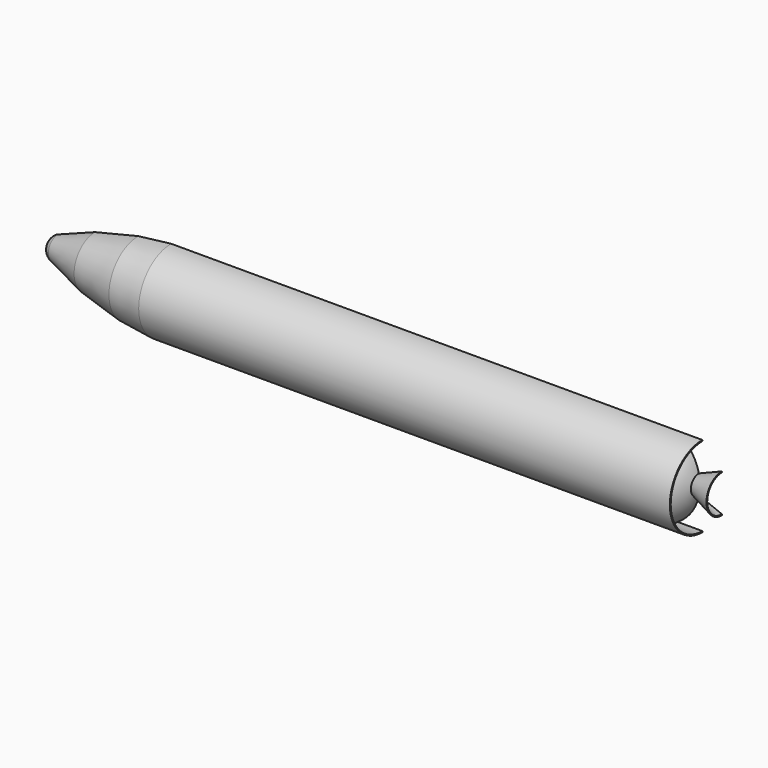
from build123d import *

# Parameters (mm, degrees)
F1_ANGLE = 180


with BuildPart() as f1:
    # F0 (on Front) → F1 (revolve)
    with BuildSketch(Plane.XZ):
        with BuildLine():
            Line((13952.3196879505, 1066.8), (0, 1066.8))
            Line((0, 1066.8), (-864.9686047513, 961.8114734625))
            Line((-864.9686047513, 961.8114734625), (-2002.3552955837, 684.0247720961))
            Line((-2002.3552955837, 684.0247720961), (-2976.9514947803, 312.9691331448))
            ThreePointArc((-2976.9514947803, 312.9691331448), (-3133.5230556351, 190.0582811283), (-3192.6803120495, 0))
            Line((-3192.6803120495, 0), (12136.4754910278, 0))
            Line((12136.4754910278, 0), (12136.4754910278, 611.6421476167))
            Line((12136.4754910278, 611.6421476167), (13157.3033463571, 611.6421476167))
            Line((13157.3033463571, 611.6421476167), (13368.401, 188.3673656228))
            ThreePointArc((13368.401, 188.3673656228), (13423.7113916071, 127.7521298206), (13502.64, 105.3084))
            ThreePointArc((13502.64, 105.3084), (13531.2627405393, 108.0644564433), (13558.8337203562, 116.2313527344))
            Line((13558.8337203562, 116.2313527344), (13952.3196879505, 275.2100031406))
            Line((13952.3196879505, 275.2100031406), (14465.935, 482.7240591992))
            Line((14465.935, 482.7240591992), (14465.935, 508))
            Line((14465.935, 508), (13860.7033572475, 263.4705436227))
            ThreePointArc((13860.7033572475, 263.4705436227), (13659.6459839666, 709.523311654), (13298.2616424561, 1039.3543243408))
            Line((13298.2616424561, 1039.3543243408), (13952.3196879505, 1039.3543243408))
            Line((13952.3196879505, 1039.3543243408), (13952.3196879505, 1066.8))
        make_face()
    revolve(axis=Axis((28212.9992331256, 0, 0), (1, 0, 0)), revolution_arc=F1_ANGLE)


solid = f1.part
